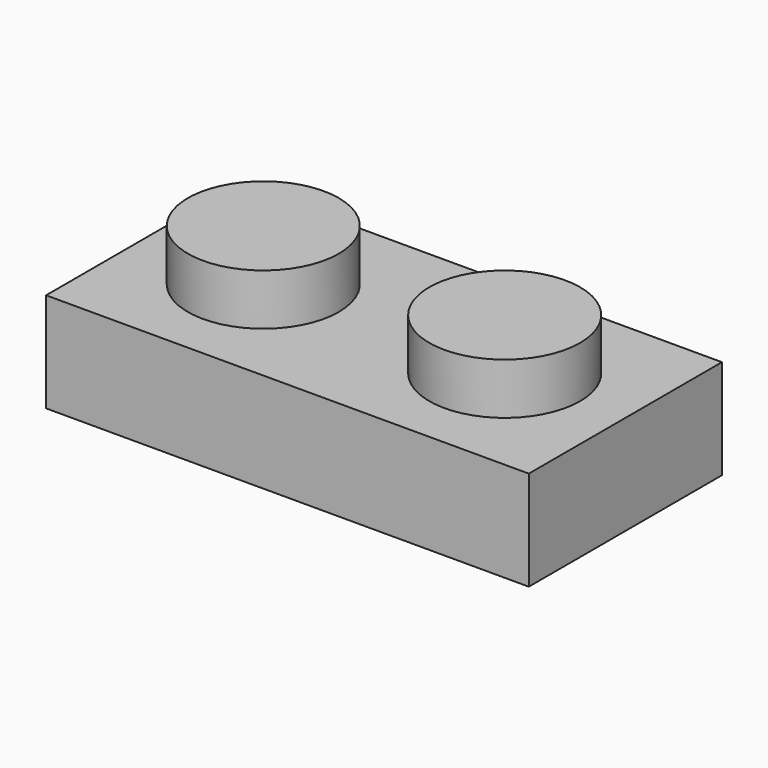
from build123d import *

# Parameters (mm, degrees)
F0_W        = 16
F0_H        = 8
F1_DEPTH    = 3.3
F3_R        = 2.5
F4_DEPTH    = 1.7
F6_T        = -1.5
F7_DEPTH    = 3.3
F8_T        = 0.8
F8_T3_DEPTH = 3.4
F8_T5_DEPTH = 6.6
F8_T7_DEPTH = 14.6


# Not quite as in the source:
# - a shell that OpenCascade refuses in one call is made with other operations: the cavity is built on its own and cut out


with BuildPart() as f1:
    # F0 (on Top) → F1 (new body)
    with BuildSketch(Plane.XY):
        with Locations((-50.3335684606, 35.747165516)):
            Rectangle(F0_W, F0_H)
    extrude(amount=F1_DEPTH)

    # F3 (on face) → F4 (join)
    with BuildSketch(Plane.XY.offset(3.3)):
        with Locations((-46.3335684606, 35.747165516)):
            Circle(F3_R)
        with Locations((-54.3335684606, 35.747165516)):
            Circle(F3_R)
    extrude(amount=F4_DEPTH)

    # F6
    f6_openings = [f1.faces().sort_by_distance(p)[0] for p in [
        (-50.333568, 35.747166, 0),
    ]]
    offset(amount=F6_T, openings=f6_openings, kind=Kind.INTERSECTION)

    # F5 (on face) → F7 (join)
    with BuildSketch(Plane.XY.offset(3.3)):
        with BuildLine():
            ThreePointArc((-51.8335684606, 35.747165516), (-50.3335684606, 34.247165516), (-48.8335684606, 35.747165516))
            ThreePointArc((-48.8335684606, 35.747165516), (-50.3335684606, 37.247165516), (-51.8335684606, 35.747165516))
        make_face()
    extrude(amount=-F7_DEPTH)

    # F8: shell of thickness 0.8, made by hand


with BuildPart() as f8_core1:
    # F8_t2: copy of F1
    add(f1.part)

    # the walls: a layer under each face that stays
    f8_faces = [f8_core1.faces().sort_by_distance(p)[0] for p in [
        (-50.3335684606, 39.747165516, 1.65),
        (-50.3335684606, 35.747165516, 3.3),
        (-48.8335684606, 35.747165516, 4.15),
        (-46.3335684606, 35.747165516, 5),
        (-56.8335684606, 35.747165516, 4.15),
        (-54.3335684606, 35.747165516, 5),
        (-50.3335684606, 31.747165516, 1.65),
        (-55.666901794, 33.0804988494, 0),
        (-56.8335684606, 35.747165516, 0.9),
        (-54.666901794, 34.0804988494, 1.8),
        (-47.3335684606, 35.747165516, 2.65),
        (-46.3335684606, 35.747165516, 3.5),
        (-48.8335684606, 35.747165516, 0.9),
        (-55.3335684606, 35.747165516, 2.65),
        (-54.3335684606, 35.747165516, 3.5),
        (-50.3335684606, 33.247165516, 0.9),
        (-43.8335684606, 35.747165516, 0.9),
        (-50.3335684606, 38.247165516, 0.9),
        (-58.3335684606, 35.747165516, 1.65),
        (-42.3335684606, 35.747165516, 1.65),
    ]]
    thicken(f8_faces, amount=-F8_T, mode=Mode.SUBTRACT)

    # F8_s4 → F8_t3 (cut)
    with BuildSketch(Plane.XY.offset(-0.8)):
        Polygon((-56.8255684606, 33.255165516), (-57.6335684606, 33.247165516), (-57.6335684606, 32.447165516), (-56.8335684606, 32.447165516), align=None)
        Polygon((-56.8255684606, 38.239165516), (-57.6335684606, 38.247165516), (-57.6335684606, 39.047165516), (-56.8335684606, 39.047165516), align=None)
        Polygon((-43.8415684606, 33.255165516), (-43.8335684606, 32.447165516), (-43.0335684606, 32.447165516), (-43.0335684606, 33.247165516), align=None)
        Polygon((-43.8415684606, 38.239165516), (-43.0335684606, 38.247165516), (-43.0335684606, 39.047165516), (-43.8335684606, 39.047165516), align=None)
    extrude(amount=F8_T3_DEPTH, mode=Mode.SUBTRACT)

    # F8_s6 → F8_t5 (cut)
    with BuildSketch(Plane.XZ.offset(-39.047165516)):
        Polygon((-56.8255684606, 1.792), (-57.6335684606, 1.8), (-57.6335684606, 2.6), (-56.8335684606, 2.6), align=None)
        Polygon((-43.8415684606, 1.792), (-43.8335684606, 2.6), (-43.0335684606, 2.6), (-43.0335684606, 1.8), align=None)
    extrude(amount=F8_T5_DEPTH, mode=Mode.SUBTRACT)

    # F8_s8 → F8_t7 (cut)
    with BuildSketch(Plane.YZ.offset(-57.6335684606)):
        Polygon((33.255165516, 1.792), (33.247165516, 2.6), (32.447165516, 2.6), (32.447165516, 1.8), align=None)
        Polygon((38.239165516, 1.792), (38.247165516, 2.6), (39.047165516, 2.6), (39.047165516, 1.8), align=None)
    extrude(amount=F8_T7_DEPTH, mode=Mode.SUBTRACT)

    # F8_s9 → F8_t10 (revolve, cut)
    with BuildSketch(Plane.XZ.offset(-35.747165516)):
        Polygon((-51.8255684606, 3.308), (-51.8335684606, 2.5), (-52.6335684606, 2.5), (-52.6335684606, 3.3), align=None)
    revolve(axis=Axis((-54.3335684606, 35.747165516, 3.3), (0, 0, 1)), mode=Mode.SUBTRACT)

    # F8_s11 → F8_t12 (revolve, cut)
    with BuildSketch(Plane.XZ.offset(-35.747165516)):
        Polygon((-43.8255684606, 3.308), (-43.8335684606, 2.5), (-44.6335684606, 2.5), (-44.6335684606, 3.3), align=None)
    revolve(axis=Axis((-46.3335684606, 35.747165516, 3.3), (0, 0, -1)), mode=Mode.SUBTRACT)

    # F8_s13 → F8_t14 (revolve, cut)
    with BuildSketch(Plane.XZ.offset(-35.747165516)):
        Polygon((-51.8415684606, 1.792), (-51.8335684606, 2.6), (-51.0335684606, 2.6), (-51.0335684606, 1.8), align=None)
    revolve(axis=Axis((-50.3335684606, 35.747165516, 1.8), (0, 0, 1)), mode=Mode.SUBTRACT)

    # F8_s15 → F8_t16 (revolve, cut)
    with BuildSketch(Plane.XZ.offset(-35.747165516)):
        Polygon((-45.3415684606, 3.492), (-44.5335684606, 3.5), (-44.5335684606, 4.3), (-45.3335684606, 4.3), align=None)
    revolve(axis=Axis((-46.3335684606, 35.747165516, 3.5), (0, 0, -1)), mode=Mode.SUBTRACT)

    # F8_s17 → F8_t18 (revolve, cut)
    with BuildSketch(Plane.XZ.offset(-35.747165516)):
        Polygon((-53.3415684606, 3.492), (-52.5335684606, 3.5), (-52.5335684606, 4.3), (-53.3335684606, 4.3), align=None)
    revolve(axis=Axis((-54.3335684606, 35.747165516, 3.5), (0, 0, -1)), mode=Mode.SUBTRACT)


with BuildPart() as f1_1:
    add(f1.part)

    # what is left inside the walls is the cavity
    f8_cavity = [f8_core1.part.solids().sort_by_distance(p)[0] for p in [
        (-49.641568, 35.747166, 1.666667),
    ]]
    add(f8_cavity, mode=Mode.SUBTRACT)


solid = f1_1.part
